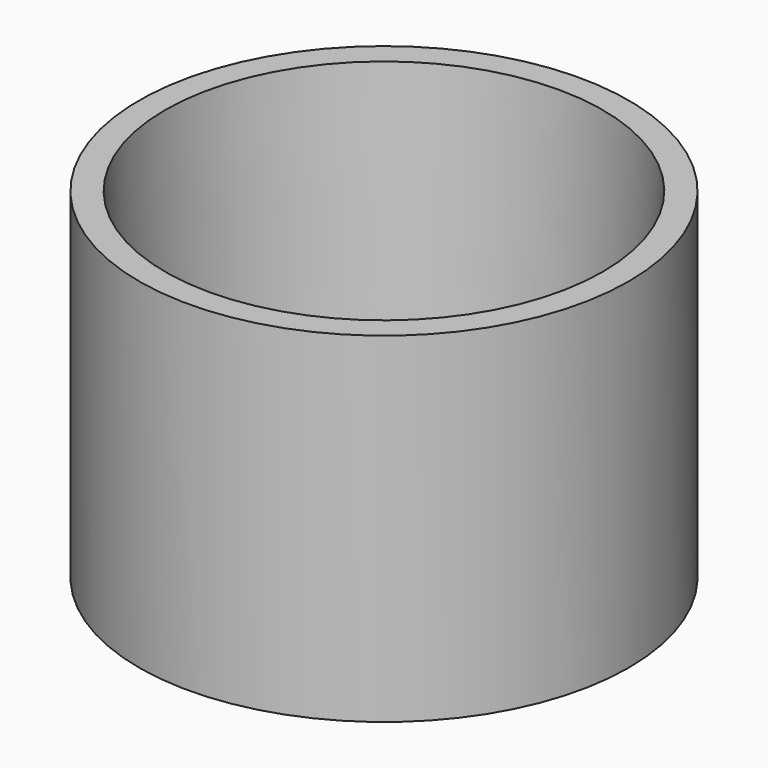
from build123d import *

# Parameters (mm, degrees)
F0_R     = 18
F0_R_2   = 15
F1_DEPTH = 25
F2_SIZE2 = 1.091514
F2_SIZE  = 24.99999
F3_W     = 11.1970370635
F3_H     = 2.7507020859
F3_W_2   = 2.8398953145
F3_H_2   = 11.1970370635
F3_H_3   = 3.1587614212
F3_W_3   = 2.980374964
F4_DEPTH = 1


# Not quite as in the source:
# - a fillet or chamfer is up to 0.001 mm smaller than in the source, because OpenCascade refuses the exact size


with BuildPart() as f1:
    # F0 (on Top) → F1 (new body)
    with BuildSketch(Plane.XY):
        Circle(F0_R)
        Circle(F0_R_2, mode=Mode.SUBTRACT)
    extrude(amount=F1_DEPTH)

    # F2 (size 25 and 1.0915235727 in the source; OpenCascade refuses exactly that, so slightly less here)
    f2_edges = [f1.edges().sort_by_distance(p)[0] for p in [
        (-15, 0, 25),
    ]]
    f2_side = f1.faces().sort_by_distance((-15, 0, 12.5))[0]
    chamfer(f2_edges, length=F2_SIZE, length2=F2_SIZE2, reference=f2_side)

    # F3 (on Top) → F4 (join)
    with BuildSketch(Plane.XY):
        with Locations((-9.9286013283, 2.9547317536)):
            Rectangle(F3_W, F3_H)
        with Locations((-9.9286013283, -2.9547317536)):
            Rectangle(F3_W, F3_H)
        with Locations((2.9101351392, 9.9286013283)):
            Rectangle(F3_W_2, F3_H_2)
        with Locations((-2.9101351392, 9.9286013283)):
            Rectangle(F3_W_2, F3_H_2)
        with Locations((9.9286013283, 2.9547317536)):
            Rectangle(F3_W, F3_H)
        with Locations((9.9286013283, -2.9547317536)):
            Rectangle(F3_W, F3_H)
        with Locations((2.9101351392, -9.9286013283)):
            Rectangle(F3_W_2, F3_H_2)
        with Locations((-2.9101351392, -9.9286013283)):
            Rectangle(F3_W_2, F3_H_2)
        with Locations((2.9101351392, 2.9547317536)):
            Rectangle(F3_W_2, F3_H)
        with Locations((-2.9101351392, 2.9547317536)):
            Rectangle(F3_W_2, F3_H)
        with Locations((-2.9101351392, 0)):
            Rectangle(F3_W_2, F3_H_3)
        with Locations((-2.9101351392, -2.9547317536)):
            Rectangle(F3_W_2, F3_H)
        with Locations((0, -2.9547317536)):
            Rectangle(F3_W_3, F3_H)
        with Locations((2.9101351392, -2.9547317536)):
            Rectangle(F3_W_2, F3_H)
        with Locations((2.9101351392, 0)):
            Rectangle(F3_W_2, F3_H_3)
        with Locations((0, 2.9547317536)):
            Rectangle(F3_W_3, F3_H)
        Rectangle(F3_W_3, F3_H_3)
    extrude(amount=F4_DEPTH)


solid = f1.part
